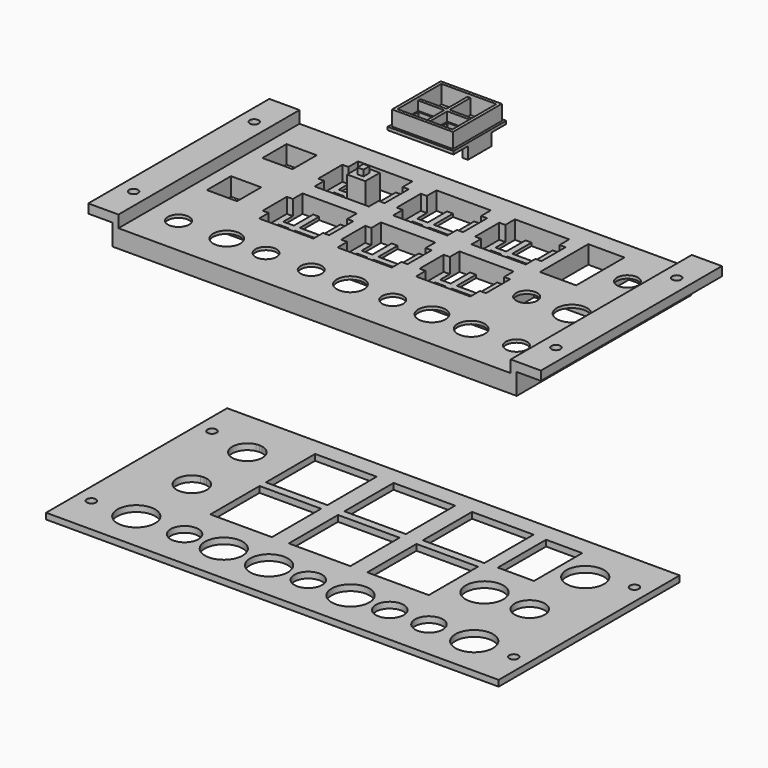
from build123d import *

# Parameters (mm, degrees)
F0_W      = 150
F0_H      = 75
F0_R      = 1.5
F0_R_2    = 3.5
F0_R_3    = 4.5
F0_R_4    = 5
F0_W_2    = 12
F0_H_2    = 20
F0_W_3    = 2
F0_H_3    = 10
F2_DEPTH  = 1
F3_DEPTH  = 5
F4_W      = 2
F4_H      = 10
F4_W_2    = 10
F5_DEPTH  = 5
F6_W      = 1.8
F6_H      = 9.8
F7_DEPTH  = 1
F8_DEPTH  = 4
F9_W      = 20.2
F9_H      = 20.2
F9_W_2    = 18.2
F9_H_2    = 18.2
F10_DEPTH = 5
F12_W     = 6
F12_H     = 4
F12_H_2   = 2
F13_DEPTH = 8
F11_W     = 8.6
F11_H     = 1
F11_W_2   = 1
F11_H_2   = 8.6
F14_DEPTH = 6
F15_W     = 18.2
F15_H     = 18.2
F16_DEPTH = 1
F18_W     = 2
F18_H     = 2.5
F19_DEPTH = 2
F20_W     = 8.6
F20_H     = 8.6
F20_W_2   = 7.6
F20_H_2   = 7.6
F21_DEPTH = 2
F17_W     = 2
F17_H     = 2.5
F22_DEPTH = 2
F23_R     = 3.5
F23_R_2   = 4.5
F23_R_3   = 5
F23_W     = 16
F23_H     = 21
F24_DEPTH = 5
F1_W      = 150
F1_H      = 75
F1_R      = 1.5
F1_R_2    = 6.25
F1_R_3    = 4.6
F1_W_2    = 20.4
F1_H_2    = 20.4
F1_R_4    = 5
F1_W_3    = 12
F1_H_3    = 20
F25_DEPTH = 2
F26_W     = 10
F26_H     = 75
F26_R     = 1.5
F27_DEPTH = 4
F28_W     = 8
F28_H     = 7
F29_DEPTH = 77.8
F30_W     = 134
F30_H     = 2.5
F31_DEPTH = 3


with BuildPart() as f2:
    # F0 (on Top) → F2 (new body)
    with BuildSketch(Plane.XY):
        with Locations((-80.504784634, -19.5405644029)):
            Rectangle(F0_W, F0_H)
        with Locations((-150.504784634, -44.5405644029)):
            Circle(F0_R, mode=Mode.SUBTRACT)
        with Locations((-136.004784634, -44.0405644029)):
            Circle(F0_R_2, mode=Mode.SUBTRACT)
        with Locations((-120.004784634, -44.0405644029)):
            Circle(F0_R_3, mode=Mode.SUBTRACT)
        with Locations((-107.004784634, -44.0405644029)):
            Circle(F0_R_2, mode=Mode.SUBTRACT)
        with Locations((-92.004784634, -44.0405644029)):
            Circle(F0_R_2, mode=Mode.SUBTRACT)
        Polygon((-131.004784634, -16.0405644029), (-131.004784634, -26.0405644029), (-135.004784634, -26.0405644029), (-137.004784634, -26.0405644029), (-141.004784634, -26.0405644029), (-141.004784634, -16.0405644029), (-137.004784634, -16.0405644029), (-135.004784634, -16.0405644029), align=None, mode=Mode.SUBTRACT)
        Polygon((-102.504784634, -22.0405644029), (-102.504784634, -30.0405644029), (-105.9770819313, -30.0405644029), (-107.9770819313, -30.0405644029), (-114.9770819313, -30.0405644029), (-116.9770819313, -30.0405644029), (-120.504784634, -30.0405644029), (-120.504784634, -22.0405644029), (-120.504784634, -20.0405644029), (-120.504784634, -12.0405644029), (-116.9770819313, -12.0405644029), (-114.9770819313, -12.0405644029), (-107.9770819313, -12.0405644029), (-105.9770819313, -12.0405644029), (-102.504784634, -12.0405644029), (-102.504784634, -20.0405644029), align=None, mode=Mode.SUBTRACT)
        Polygon((-76.504784634, -12.0405644029), (-76.504784634, -20.0405644029), (-76.504784634, -22.0405644029), (-76.504784634, -30.0405644029), (-79.9770819313, -30.0405644029), (-81.9770819313, -30.0405644029), (-88.9770819313, -30.0405644029), (-90.9770819313, -30.0405644029), (-94.504784634, -30.0405644029), (-94.504784634, -22.0405644029), (-94.504784634, -20.0405644029), (-94.504784634, -12.0405644029), (-90.9770819313, -12.0405644029), (-88.9770819313, -12.0405644029), (-81.9770819313, -12.0405644029), (-79.9770819313, -12.0405644029), align=None, mode=Mode.SUBTRACT)
        with Locations((-79.004784634, -44.0405644029)):
            Circle(F0_R_3, mode=Mode.SUBTRACT)
        with Locations((-65.004784634, -44.0405644029)):
            Circle(F0_R_2, mode=Mode.SUBTRACT)
        with Locations((-52.004784634, -44.0405644029)):
            Circle(F0_R_3, mode=Mode.SUBTRACT)
        with Locations((-39.004784634, -44.0405644029)):
            Circle(F0_R_3, mode=Mode.SUBTRACT)
        with Locations((-24.004784634, -44.0405644029)):
            Circle(F0_R_2, mode=Mode.SUBTRACT)
        with Locations((-10.504784634, -44.5405644029)):
            Circle(F0_R, mode=Mode.SUBTRACT)
        Polygon((-50.504784634, -12.0405644029), (-50.504784634, -20.0405644029), (-50.504784634, -22.0405644029), (-50.504784634, -30.0405644029), (-53.9770819313, -30.0405644029), (-55.9770819313, -30.0405644029), (-62.9770819313, -30.0405644029), (-64.9770819313, -30.0405644029), (-68.504784634, -30.0405644029), (-68.504784634, -22.0405644029), (-68.504784634, -20.0405644029), (-68.504784634, -12.0405644029), (-64.9770819313, -12.0405644029), (-62.9770819313, -12.0405644029), (-55.9770819313, -12.0405644029), (-53.9770819313, -12.0405644029), align=None, mode=Mode.SUBTRACT)
        with Locations((-39.004784634, -21.0405644029)):
            Circle(F0_R_2, mode=Mode.SUBTRACT)
        with Locations((-24.004784634, -21.0405644029)):
            Circle(F0_R_4, mode=Mode.SUBTRACT)
        with Locations((-150.504784634, 5.4594355971)):
            Circle(F0_R, mode=Mode.SUBTRACT)
        Polygon((-131.004784634, 6.9594355971), (-131.004784634, -3.0405644029), (-135.004784634, -3.0405644029), (-137.004784634, -3.0405644029), (-141.004784634, -3.0405644029), (-141.004784634, 6.9594355971), (-137.004784634, 6.9594355971), (-135.004784634, 6.9594355971), align=None, mode=Mode.SUBTRACT)
        Polygon((-102.504784634, 0.9594355971), (-102.504784634, -7.0405644029), (-106.004784634, -7.0405644029), (-108.004784634, -7.0405644029), (-115.004784634, -7.0405644029), (-117.004784634, -7.0405644029), (-120.504784634, -7.0405644029), (-120.504784634, 0.9594355971), (-120.504784634, 2.9594355971), (-120.504784634, 10.9594355971), (-117.004784634, 10.9594355971), (-115.004784634, 10.9594355971), (-108.004784634, 10.9594355971), (-106.004784634, 10.9594355971), (-102.504784634, 10.9594355971), (-102.504784634, 2.9594355971), align=None, mode=Mode.SUBTRACT)
        Polygon((-94.504784634, 10.9594355971), (-91.004784634, 10.9594355971), (-89.004784634, 10.9594355971), (-82.004784634, 10.9594355971), (-80.004784634, 10.9594355971), (-76.504784634, 10.9594355971), (-76.504784634, 2.9594355971), (-76.504784634, 0.9594355971), (-76.504784634, -7.0405644029), (-80.004784634, -7.0405644029), (-82.004784634, -7.0405644029), (-89.004784634, -7.0405644029), (-91.004784634, -7.0405644029), (-94.504784634, -7.0405644029), (-94.504784634, 0.9594355971), (-94.504784634, 2.9594355971), align=None, mode=Mode.SUBTRACT)
        Polygon((-68.504784634, 10.9594355971), (-65.004784634, 10.9594355971), (-63.004784634, 10.9594355971), (-56.004784634, 10.9594355971), (-54.004784634, 10.9594355971), (-50.504784634, 10.9594355971), (-50.504784634, 2.9594355971), (-50.504784634, 0.9594355971), (-50.504784634, -7.0405644029), (-54.004784634, -7.0405644029), (-56.004784634, -7.0405644029), (-63.004784634, -7.0405644029), (-65.004784634, -7.0405644029), (-68.504784634, -7.0405644029), (-68.504784634, 0.9594355971), (-68.504784634, 2.9594355971), align=None, mode=Mode.SUBTRACT)
        with Locations((-39.004784634, 1.9594355971)):
            Rectangle(F0_W_2, F0_H_2, mode=Mode.SUBTRACT)
        with Locations((-24.004784634, 1.9594355971)):
            Circle(F0_R_2, mode=Mode.SUBTRACT)
        with Locations((-10.504784634, 5.4594355971)):
            Circle(F0_R, mode=Mode.SUBTRACT)
        Polygon((-108.004784634, -7.0405644029), (-106.004784634, -7.0405644029), (-106.004784634, 0.9594355971), (-102.504784634, 0.9594355971), (-102.504784634, 2.9594355971), (-106.004784634, 2.9594355971), (-106.004784634, 10.9594355971), (-108.004784634, 10.9594355971), (-108.004784634, 2.9594355971), (-115.004784634, 2.9594355971), (-115.004784634, 10.9594355971), (-117.004784634, 10.9594355971), (-117.004784634, 2.9594355971), (-120.504784634, 2.9594355971), (-120.504784634, 0.9594355971), (-117.004784634, 0.9594355971), (-117.004784634, -7.0405644029), (-115.004784634, -7.0405644029), (-115.004784634, 0.9594355971), (-108.004784634, 0.9594355971), align=None)
        Polygon((-107.9770819313, -30.0405644029), (-105.9770819313, -30.0405644029), (-105.9770819313, -22.0405644029), (-102.504784634, -22.0405644029), (-102.504784634, -20.0405644029), (-105.9770819313, -20.0405644029), (-105.9770819313, -12.0405644029), (-107.9770819313, -12.0405644029), (-107.9770819313, -20.0405644029), (-114.9770819313, -20.0405644029), (-114.9770819313, -12.0405644029), (-116.9770819313, -12.0405644029), (-116.9770819313, -20.0405644029), (-120.504784634, -20.0405644029), (-120.504784634, -22.0405644029), (-116.9770819313, -22.0405644029), (-116.9770819313, -30.0405644029), (-114.9770819313, -30.0405644029), (-114.9770819313, -22.0405644029), (-107.9770819313, -22.0405644029), align=None)
        Polygon((-91.004784634, 10.9594355971), (-91.004784634, 2.9594355971), (-94.504784634, 2.9594355971), (-94.504784634, 0.9594355971), (-91.004784634, 0.9594355971), (-91.004784634, -7.0405644029), (-89.004784634, -7.0405644029), (-89.004784634, 0.9594355971), (-82.004784634, 0.9594355971), (-82.004784634, -7.0405644029), (-80.004784634, -7.0405644029), (-80.004784634, 0.9594355971), (-76.504784634, 0.9594355971), (-76.504784634, 2.9594355971), (-80.004784634, 2.9594355971), (-80.004784634, 10.9594355971), (-82.004784634, 10.9594355971), (-82.004784634, 2.9594355971), (-89.004784634, 2.9594355971), (-89.004784634, 10.9594355971), align=None)
        Polygon((-65.004784634, 10.9594355971), (-65.004784634, 2.9594355971), (-68.504784634, 2.9594355971), (-68.504784634, 0.9594355971), (-65.004784634, 0.9594355971), (-65.004784634, -7.0405644029), (-63.004784634, -7.0405644029), (-63.004784634, 0.9594355971), (-56.004784634, 0.9594355971), (-56.004784634, -7.0405644029), (-54.004784634, -7.0405644029), (-54.004784634, 0.9594355971), (-50.504784634, 0.9594355971), (-50.504784634, 2.9594355971), (-54.004784634, 2.9594355971), (-54.004784634, 10.9594355971), (-56.004784634, 10.9594355971), (-56.004784634, 2.9594355971), (-63.004784634, 2.9594355971), (-63.004784634, 10.9594355971), align=None)
        Polygon((-50.504784634, -22.0405644029), (-50.504784634, -20.0405644029), (-53.9770819313, -20.0405644029), (-53.9770819313, -12.0405644029), (-55.9770819313, -12.0405644029), (-55.9770819313, -20.0405644029), (-62.9770819313, -20.0405644029), (-62.9770819313, -12.0405644029), (-64.9770819313, -12.0405644029), (-64.9770819313, -20.0405644029), (-68.504784634, -20.0405644029), (-68.504784634, -22.0405644029), (-64.9770819313, -22.0405644029), (-64.9770819313, -30.0405644029), (-62.9770819313, -30.0405644029), (-62.9770819313, -22.0405644029), (-55.9770819313, -22.0405644029), (-55.9770819313, -30.0405644029), (-53.9770819313, -30.0405644029), (-53.9770819313, -22.0405644029), align=None)
        Polygon((-76.504784634, -22.0405644029), (-76.504784634, -20.0405644029), (-79.9770819313, -20.0405644029), (-79.9770819313, -12.0405644029), (-81.9770819313, -12.0405644029), (-81.9770819313, -20.0405644029), (-88.9770819313, -20.0405644029), (-88.9770819313, -12.0405644029), (-90.9770819313, -12.0405644029), (-90.9770819313, -20.0405644029), (-94.504784634, -20.0405644029), (-94.504784634, -22.0405644029), (-90.9770819313, -22.0405644029), (-90.9770819313, -30.0405644029), (-88.9770819313, -30.0405644029), (-88.9770819313, -22.0405644029), (-81.9770819313, -22.0405644029), (-81.9770819313, -30.0405644029), (-79.9770819313, -30.0405644029), (-79.9770819313, -22.0405644029), align=None)
        with Locations((-136.004784634, 1.9594355971)):
            Rectangle(F0_W_3, F0_H_3)
        with Locations((-136.004784634, -21.0405644029)):
            Rectangle(F0_W_3, F0_H_3)
    extrude(amount=F2_DEPTH)

    # F3 (add): a face of the model
    f3_faces = [f2.faces().sort_by_distance(p)[0] for p in [
        (-80.9297828896, -20.6563587059, 1),
    ]]
    extrude(f3_faces, amount=F3_DEPTH)

    # F4 (on face) → F5 (cut)
    with BuildSketch(Plane.XY.offset(6)):
        Polygon((-120.504784634, -7.0405644029), (-102.504784634, -7.0405644029), (-102.504784634, -3.0405644029), (-102.504784634, 6.9594355971), (-102.504784634, 10.9594355971), (-120.504784634, 10.9594355971), (-120.504784634, 6.9594355971), (-120.504784634, -3.0405644029), align=None)
        with Locations((-101.504784634, 1.9594355971)):
            Rectangle(F4_W, F4_H)
        with Locations((-121.504784634, 1.9594355971)):
            Rectangle(F4_W, F4_H)
        Polygon((-120.504784634, -30.0405644029), (-102.504784634, -30.0405644029), (-102.504784634, -26.0405644029), (-102.504784634, -16.0405644029), (-102.504784634, -12.0405644029), (-120.504784634, -12.0405644029), (-120.504784634, -16.0405644029), (-120.504784634, -26.0405644029), align=None)
        with Locations((-101.504784634, -21.0405644029)):
            Rectangle(F4_W, F4_H)
        with Locations((-121.504784634, -21.0405644029)):
            Rectangle(F4_W, F4_H)
        with Locations((-75.504784634, 1.9594355971)):
            Rectangle(F4_W, F4_H)
        Polygon((-76.504784634, -7.0405644029), (-76.504784634, -3.0405644029), (-76.504784634, 6.9594355971), (-76.504784634, 10.9594355971), (-94.504784634, 10.9594355971), (-94.504784634, 6.9594355971), (-94.504784634, -3.0405644029), (-94.504784634, -7.0405644029), align=None)
        with Locations((-95.504784634, 1.9594355971)):
            Rectangle(F4_W, F4_H)
        with Locations((-49.504784634, 1.9594355971)):
            Rectangle(F4_W, F4_H)
        Polygon((-50.504784634, -7.0405644029), (-50.504784634, -3.0405644029), (-50.504784634, 6.9594355971), (-50.504784634, 10.9594355971), (-68.504784634, 10.9594355971), (-68.504784634, 6.9594355971), (-68.504784634, -3.0405644029), (-68.504784634, -7.0405644029), align=None)
        with Locations((-69.504784634, 1.9594355971)):
            Rectangle(F4_W, F4_H)
        with Locations((-75.504784634, -21.0405644029)):
            Rectangle(F4_W, F4_H)
        Polygon((-76.504784634, -26.0405644029), (-76.504784634, -16.0405644029), (-76.504784634, -12.0405644029), (-94.504784634, -12.0405644029), (-94.504784634, -16.0405644029), (-94.504784634, -26.0405644029), (-94.504784634, -30.0405644029), (-76.504784634, -30.0405644029), align=None)
        with Locations((-95.504784634, -21.0405644029)):
            Rectangle(F4_W, F4_H)
        with Locations((-49.504784634, -21.0405644029)):
            Rectangle(F4_W, F4_H)
        Polygon((-50.504784634, -26.0405644029), (-50.504784634, -16.0405644029), (-50.504784634, -12.0405644029), (-68.504784634, -12.0405644029), (-68.504784634, -16.0405644029), (-68.504784634, -26.0405644029), (-68.504784634, -30.0405644029), (-50.504784634, -30.0405644029), align=None)
        with Locations((-69.504784634, -21.0405644029)):
            Rectangle(F4_W, F4_H)
        with Locations((-136.004784634, 1.9594355971)):
            Rectangle(F4_W_2, F4_H)
        with Locations((-136.004784634, -21.0405644029)):
            Rectangle(F4_W_2, F4_H)
    extrude(amount=-F5_DEPTH, mode=Mode.SUBTRACT)

    # F12 (on face) → F13 (join)
    with BuildSketch(Plane.XY.offset(1)):
        with Locations((-111.504784634, 2.9594355971)):
            Rectangle(F12_W, F12_H)
        with Locations((-111.504784634, -0.0405644029)):
            Rectangle(F12_W, F12_H_2)
    extrude(amount=F13_DEPTH)

    # F18 (on face) → F19 (join)
    with BuildSketch(Plane.XY.offset(9)):
        with Locations((-111.504784634, 1.9594355971)):
            Rectangle(F18_W, F18_H)
    extrude(amount=F19_DEPTH)

    # F23 (on face) → F24 (cut)
    with BuildSketch(Plane.XY):
        Polygon((-44.504784634, -33.0405644029), (-145.504784634, -33.0405644029), (-145.504784634, -55.0405644029), (-15.504784634, -55.0405644029), (-15.504784634, -33.0405644029), align=None)
        with Locations((-136.004784634, -44.0405644029)):
            Circle(F23_R, mode=Mode.SUBTRACT)
        with Locations((-120.004784634, -44.0405644029)):
            Circle(F23_R_2, mode=Mode.SUBTRACT)
        with Locations((-107.004784634, -44.0405644029)):
            Circle(F23_R, mode=Mode.SUBTRACT)
        with Locations((-92.004784634, -44.0405644029)):
            Circle(F23_R, mode=Mode.SUBTRACT)
        with Locations((-79.004784634, -44.0405644029)):
            Circle(F23_R_2, mode=Mode.SUBTRACT)
        with Locations((-65.004784634, -44.0405644029)):
            Circle(F23_R, mode=Mode.SUBTRACT)
        with Locations((-52.004784634, -44.0405644029)):
            Circle(F23_R_2, mode=Mode.SUBTRACT)
        with Locations((-39.004784634, -44.0405644029)):
            Circle(F23_R_2, mode=Mode.SUBTRACT)
        with Locations((-24.004784634, -44.0405644029)):
            Circle(F23_R, mode=Mode.SUBTRACT)
        Polygon((-44.504784634, -11.0405644029), (-44.504784634, -31.0405644029), (-15.504784634, -31.0405644029), (-15.504784634, -11.0405644029), (-31.504784634, -11.0405644029), align=None)
        with Locations((-39.004784634, -21.0405644029)):
            Circle(F23_R, mode=Mode.SUBTRACT)
        with Locations((-24.004784634, -21.0405644029)):
            Circle(F23_R_3, mode=Mode.SUBTRACT)
        with Locations((-23.504784634, 1.4594355971)):
            Rectangle(F23_W, F23_H)
        with Locations((-24.004784634, 1.9594355971)):
            Circle(F23_R, mode=Mode.SUBTRACT)
        with Locations((-24.004784634, -21.0405644029)):
            Circle(F23_R_3)
        with Locations((-120.004784634, -44.0405644029)):
            Circle(F23_R_2)
        with Locations((-79.004784634, -44.0405644029)):
            Circle(F23_R_2)
        with Locations((-52.004784634, -44.0405644029)):
            Circle(F23_R_2)
        with Locations((-39.004784634, -44.0405644029)):
            Circle(F23_R_2)
        with Locations((-136.004784634, -44.0405644029)):
            Circle(F23_R)
        with Locations((-107.004784634, -44.0405644029)):
            Circle(F23_R)
        with Locations((-92.004784634, -44.0405644029)):
            Circle(F23_R)
        with Locations((-65.004784634, -44.0405644029)):
            Circle(F23_R)
        with Locations((-24.004784634, -44.0405644029)):
            Circle(F23_R)
        with Locations((-39.004784634, -21.0405644029)):
            Circle(F23_R)
        with Locations((-24.004784634, 1.9594355971)):
            Circle(F23_R)
    extrude(amount=F24_DEPTH, mode=Mode.SUBTRACT)

    # F26 (on face) → F27 (join)
    with BuildSketch(Plane.XY.offset(6)):
        with Locations((-10.504784634, -19.5405644029)):
            Rectangle(F26_W, F26_H)
        with Locations((-10.504784634, -44.5405644029)):
            Circle(F26_R, mode=Mode.SUBTRACT)
        with Locations((-10.504784634, 5.4594355971)):
            Circle(F26_R, mode=Mode.SUBTRACT)
        with Locations((-150.504784634, -19.5405644029)):
            Rectangle(F26_W, F26_H)
        with Locations((-150.504784634, -44.5405644029)):
            Circle(F26_R, mode=Mode.SUBTRACT)
        with Locations((-150.504784634, 5.4594355971)):
            Circle(F26_R, mode=Mode.SUBTRACT)
    extrude(amount=F27_DEPTH)

    # F28 (on face) → F29 (cut)
    with BuildSketch(Plane.XZ.offset(57.0405644029)):
        with Locations((-151.504784634, 3.5)):
            Rectangle(F28_W, F28_H)
        with Locations((-9.504784634, 3.5)):
            Rectangle(F28_W, F28_H)
    extrude(amount=-F29_DEPTH, mode=Mode.SUBTRACT)

    # F30 (on face) → F31 (cut)
    with BuildSketch(Plane(origin=(0, 0, 0), x_dir=(1, 0, 0), z_dir=(0, 0, -1))):
        with Locations((-80.504784634, -16.7094355971)):
            Rectangle(F30_W, F30_H)
    extrude(amount=-F31_DEPTH, mode=Mode.SUBTRACT)


with BuildPart() as f7:
    # F6 (on Top) → F7 (new body)
    with BuildSketch(Plane.XY):
        Polygon((-132.6183355093, 38.3936729491), (-110.8183355093, 38.3936729491), (-110.8183355093, 44.3936729491), (-112.6183355093, 44.3936729491), (-112.6183355093, 40.1936729491), (-130.8183355093, 40.1936729491), (-130.8183355093, 44.3936729491), (-132.6183355093, 44.3936729491), align=None)
        with Locations((-111.7183355093, 49.2936729491)):
            Rectangle(F6_W, F6_H)
        with Locations((-131.7183355093, 49.2936729491)):
            Rectangle(F6_W, F6_H)
        Polygon((-112.6183355093, 54.1936729491), (-110.8183355093, 54.1936729491), (-110.8183355093, 60.1936729491), (-132.6183355093, 60.1936729491), (-132.6183355093, 54.1936729491), (-130.8183355093, 54.1936729491), (-130.8183355093, 58.3936729491), (-112.6183355093, 58.3936729491), align=None)
    extrude(amount=F7_DEPTH)

    # F6 (on Top) → F8 (join)
    with BuildSketch(Plane.XY):
        with Locations((-131.7183355093, 49.2936729491)):
            Rectangle(F6_W, F6_H)
        with Locations((-111.7183355093, 49.2936729491)):
            Rectangle(F6_W, F6_H)
    extrude(amount=-F8_DEPTH)

    # F9 (on face) → F10 (join)
    with BuildSketch(Plane.XY.offset(1)):
        with Locations((-121.7183355093, 49.2936729491)):
            Rectangle(F9_W, F9_H)
        with Locations((-121.7183355093, 49.2936729491)):
            Rectangle(F9_W_2, F9_H_2, mode=Mode.SUBTRACT)
    extrude(amount=F10_DEPTH)

    # F11 (on face) → F14 (join)
    with BuildSketch(Plane.XY.offset(6)):
        with Locations((-116.9183355093, 49.2936729491)):
            Rectangle(F11_W, F11_H)
        with Locations((-121.7183355093, 44.4936729491)):
            Rectangle(F11_W_2, F11_H_2)
        with Locations((-121.7183355093, 49.2936729491)):
            Rectangle(F11_W_2, F11_H)
        with Locations((-126.5183355093, 49.2936729491)):
            Rectangle(F11_W, F11_H)
        with Locations((-121.7183355093, 54.0936729491)):
            Rectangle(F11_W_2, F11_H_2)
    extrude(amount=-F14_DEPTH)

    # F15 (on face) → F16 (cut)
    with BuildSketch(Plane.XY.offset(6)):
        with Locations((-121.7183355093, 49.2936729491)):
            Rectangle(F15_W, F15_H)
    extrude(amount=-F16_DEPTH, mode=Mode.SUBTRACT)

    # F20 (on face) → F21 (join)
    with BuildSketch(Plane(origin=(0, 0, 0), x_dir=(1, 0, 0), z_dir=(0, 0, -1))):
        with Locations((-126.5183355093, -44.4936729491)):
            Rectangle(F20_W, F20_H)
        with Locations((-126.5183355093, -44.4936729491)):
            Rectangle(F20_W_2, F20_H_2, mode=Mode.SUBTRACT)
        with Locations((-116.9183355093, -44.4936729491)):
            Rectangle(F20_W, F20_H)
        with Locations((-116.9183355093, -44.4936729491)):
            Rectangle(F20_W_2, F20_H_2, mode=Mode.SUBTRACT)
    extrude(amount=-F21_DEPTH)

    # F17 (on face) → F22 (cut)
    with BuildSketch(Plane(origin=(0, 0, 0), x_dir=(1, 0, 0), z_dir=(0, 0, -1))):
        with Locations((-121.7183355093, -49.2936729491)):
            Rectangle(F17_W, F17_H)
    extrude(amount=-F22_DEPTH, mode=Mode.SUBTRACT)


with BuildPart() as f25:
    # F1 (on Top) → F25 (new body)
    with BuildSketch(Plane.XY):
        with Locations((9.6568725579, -149.7262832487)):
            Rectangle(F1_W, F1_H)
        with Locations((-60.3431274421, -174.7262832487)):
            Circle(F1_R, mode=Mode.SUBTRACT)
        with Locations((-45.8431274421, -174.2262832487)):
            Circle(F1_R_2, mode=Mode.SUBTRACT)
        with Locations((-29.8431274421, -174.2262832487)):
            Circle(F1_R_3, mode=Mode.SUBTRACT)
        with Locations((-16.8431274421, -174.2262832487)):
            Circle(F1_R_2, mode=Mode.SUBTRACT)
        with Locations((-1.8431274421, -174.2262832487)):
            Circle(F1_R_2, mode=Mode.SUBTRACT)
        with BuildLine():
            Line((-44.8431274421, -156.1252627342), (-44.8431274421, -156.2262832487))
            Line((-44.8431274421, -156.2262832487), (-45.8431274421, -156.2262832487))
            Line((-45.8431274421, -156.2262832487), (-46.8431274421, -156.2262832487))
            Line((-46.8431274421, -156.2262832487), (-46.8431274421, -156.1252627342))
            ThreePointArc((-46.8431274421, -156.1252627342), (-50.8431274421, -151.2262832487), (-46.8431274421, -146.3273037631))
            Line((-46.8431274421, -146.3273037631), (-46.8431274421, -146.2262832487))
            Line((-46.8431274421, -146.2262832487), (-45.8431274421, -146.2262832487))
            Line((-45.8431274421, -146.2262832487), (-44.8431274421, -146.2262832487))
            Line((-44.8431274421, -146.2262832487), (-44.8431274421, -146.3273037631))
            ThreePointArc((-44.8431274421, -146.3273037631), (-41.9701440959, -148.0640055885), (-40.8431274421, -151.2262832487))
            ThreePointArc((-40.8431274421, -151.2262832487), (-41.9701440959, -154.3885609088), (-44.8431274421, -156.1252627342))
        make_face(mode=Mode.SUBTRACT)
        with Locations((-21.3431274421, -151.2262832487)):
            Rectangle(F1_W_2, F1_H_2, mode=Mode.SUBTRACT)
        with Locations((4.6568725579, -151.2262832487)):
            Rectangle(F1_W_2, F1_H_2, mode=Mode.SUBTRACT)
        with Locations((11.1568725579, -174.2262832487)):
            Circle(F1_R_3, mode=Mode.SUBTRACT)
        with Locations((25.1568725579, -174.2262832487)):
            Circle(F1_R_2, mode=Mode.SUBTRACT)
        with Locations((38.1568725579, -174.2262832487)):
            Circle(F1_R_3, mode=Mode.SUBTRACT)
        with Locations((51.1568725579, -174.2262832487)):
            Circle(F1_R_3, mode=Mode.SUBTRACT)
        with Locations((66.1568725579, -174.2262832487)):
            Circle(F1_R_2, mode=Mode.SUBTRACT)
        with Locations((79.6568725579, -174.7262832487)):
            Circle(F1_R, mode=Mode.SUBTRACT)
        with Locations((30.6568725579, -151.2262832487)):
            Rectangle(F1_W_2, F1_H_2, mode=Mode.SUBTRACT)
        with Locations((51.1568725579, -151.2262832487)):
            Circle(F1_R_2, mode=Mode.SUBTRACT)
        with Locations((66.1568725579, -151.2262832487)):
            Circle(F1_R_4, mode=Mode.SUBTRACT)
        with Locations((-60.3431274421, -124.7262832487)):
            Circle(F1_R, mode=Mode.SUBTRACT)
        with BuildLine():
            Line((-44.8431274421, -133.1252627342), (-44.8431274421, -133.2262832487))
            Line((-44.8431274421, -133.2262832487), (-45.8431274421, -133.2262832487))
            Line((-45.8431274421, -133.2262832487), (-46.8431274421, -133.2262832487))
            Line((-46.8431274421, -133.2262832487), (-46.8431274421, -133.1252627342))
            ThreePointArc((-46.8431274421, -133.1252627342), (-50.8431274421, -128.2262832487), (-46.8431274421, -123.3273037631))
            Line((-46.8431274421, -123.3273037631), (-46.8431274421, -123.2262832487))
            Line((-46.8431274421, -123.2262832487), (-45.8431274421, -123.2262832487))
            Line((-45.8431274421, -123.2262832487), (-44.8431274421, -123.2262832487))
            Line((-44.8431274421, -123.2262832487), (-44.8431274421, -123.3273037631))
            ThreePointArc((-44.8431274421, -123.3273037631), (-41.9701440959, -125.0640055885), (-40.8431274421, -128.2262832487))
            ThreePointArc((-40.8431274421, -128.2262832487), (-41.9701440959, -131.3885609088), (-44.8431274421, -133.1252627342))
        make_face(mode=Mode.SUBTRACT)
        with Locations((-21.3431274421, -128.2262832487)):
            Rectangle(F1_W_2, F1_H_2, mode=Mode.SUBTRACT)
        with Locations((4.6568725579, -128.2262832487)):
            Rectangle(F1_W_2, F1_H_2, mode=Mode.SUBTRACT)
        with Locations((30.6568725579, -128.2262832487)):
            Rectangle(F1_W_2, F1_H_2, mode=Mode.SUBTRACT)
        with Locations((51.1568725579, -128.2262832487)):
            Rectangle(F1_W_3, F1_H_3, mode=Mode.SUBTRACT)
        with Locations((66.1568725579, -128.2262832487)):
            Circle(F1_R_2, mode=Mode.SUBTRACT)
        with Locations((79.6568725579, -124.7262832487)):
            Circle(F1_R, mode=Mode.SUBTRACT)
        with BuildLine():
            Line((-46.8431274421, -146.2262832487), (-46.8431274421, -146.3273037631))
            ThreePointArc((-46.8431274421, -146.3273037631), (-46.3456722522, -146.2516024836), (-45.8431274421, -146.2262832487))
            Line((-45.8431274421, -146.2262832487), (-46.8431274421, -146.2262832487))
        make_face()
        with BuildLine():
            ThreePointArc((-45.8431274421, -146.2262832487), (-45.3405826321, -146.2516024836), (-44.8431274421, -146.3273037631))
            Line((-44.8431274421, -146.3273037631), (-44.8431274421, -146.2262832487))
            Line((-44.8431274421, -146.2262832487), (-45.8431274421, -146.2262832487))
        make_face()
        with BuildLine():
            Line((-46.8431274421, -156.2262832487), (-45.8431274421, -156.2262832487))
            ThreePointArc((-45.8431274421, -156.2262832487), (-46.3456722522, -156.2009640137), (-46.8431274421, -156.1252627342))
            Line((-46.8431274421, -156.1252627342), (-46.8431274421, -156.2262832487))
        make_face()
        with BuildLine():
            Line((-45.8431274421, -156.2262832487), (-44.8431274421, -156.2262832487))
            Line((-44.8431274421, -156.2262832487), (-44.8431274421, -156.1252627342))
            ThreePointArc((-44.8431274421, -156.1252627342), (-45.3405826321, -156.2009640137), (-45.8431274421, -156.2262832487))
        make_face()
        with BuildLine():
            Line((-46.8431274421, -123.2262832487), (-46.8431274421, -123.3273037631))
            ThreePointArc((-46.8431274421, -123.3273037631), (-46.3456722522, -123.2516024836), (-45.8431274421, -123.2262832487))
            Line((-45.8431274421, -123.2262832487), (-46.8431274421, -123.2262832487))
        make_face()
        with BuildLine():
            ThreePointArc((-45.8431274421, -123.2262832487), (-45.3405826321, -123.2516024836), (-44.8431274421, -123.3273037631))
            Line((-44.8431274421, -123.3273037631), (-44.8431274421, -123.2262832487))
            Line((-44.8431274421, -123.2262832487), (-45.8431274421, -123.2262832487))
        make_face()
        with BuildLine():
            Line((-46.8431274421, -133.2262832487), (-45.8431274421, -133.2262832487))
            ThreePointArc((-45.8431274421, -133.2262832487), (-46.3456722522, -133.2009640137), (-46.8431274421, -133.1252627342))
            Line((-46.8431274421, -133.1252627342), (-46.8431274421, -133.2262832487))
        make_face()
        with BuildLine():
            Line((-45.8431274421, -133.2262832487), (-44.8431274421, -133.2262832487))
            Line((-44.8431274421, -133.2262832487), (-44.8431274421, -133.1252627342))
            ThreePointArc((-44.8431274421, -133.1252627342), (-45.3405826321, -133.2009640137), (-45.8431274421, -133.2262832487))
        make_face()
    extrude(amount=F25_DEPTH)


solid = Compound([f2.part, f7.part, f25.part])
